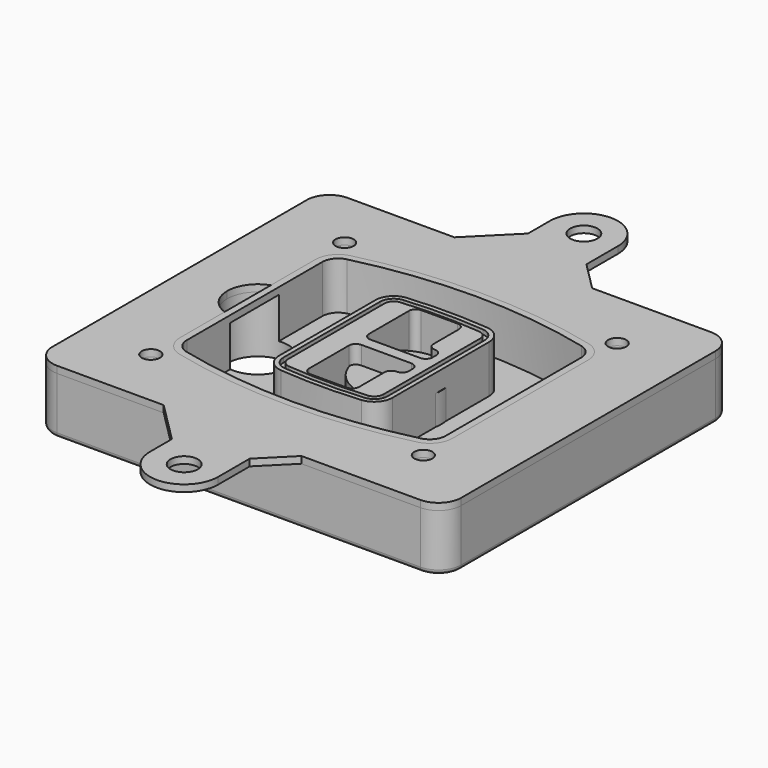
from build123d import *

# Parameters (mm, degrees)
F0_R      = 4
F1_DEPTH  = 25
F2_DEPTH  = 3
F3_DEPTH  = 18
F5_DEPTH  = 21
F6_DEPTH  = 2
F8_DEPTH  = 20
F9_DEPTH  = 16
F10_DEPTH = 25
F7_R      = 6
F7_R_2    = 4
F11_DEPTH = 6
F13_DEPTH = 9
F15_R     = 2
F16_R     = 6
F16_R_2   = 4
F17_DEPTH = 3


# Not quite as in the source:
# - a feature of the source that left no trace in its solid (it failed there, or was rolled back) is left out
# - a feature names something its author has since deleted; it is built from what else it names


with BuildPart() as f1:
    # F0 (on Top) → F1 (new body)
    with BuildSketch(Plane.XY):
        with BuildLine():
            ThreePointArc((-90, -70), (-87.0710678119, -77.0710678119), (-80, -80))
            Line((-80, -80), (80, -80))
            ThreePointArc((80, -80), (87.0710678119, -77.0710678119), (90, -70))
            Line((90, -70), (90, 70))
            ThreePointArc((90, 70), (87.0710678119, 77.0710678119), (80, 80))
            Line((80, 80), (-80, 80))
            ThreePointArc((-80, 80), (-87.0710678119, 77.0710678119), (-90, 70))
            Line((-90, 70), (-90, -70))
        make_face()
        with Locations((-60, -53.3333333333)):
            Circle(F0_R, mode=Mode.SUBTRACT)
        with Locations((60, -53.3333333333)):
            Circle(F0_R, mode=Mode.SUBTRACT)
        with Locations((-60, 53.3333333333)):
            Circle(F0_R, mode=Mode.SUBTRACT)
        with BuildLine():
            ThreePointArc((-64, 37.2990447398), (-61.0143011354, 45.9411029726), (-53.3306899286, 50.8970778549))
            ThreePointArc((-53.3306899286, 50.8970778549), (0, 57.3333333333), (53.3306899286, 50.8970778549))
            ThreePointArc((53.3306899286, 50.8970778549), (61.0143011354, 45.9411029726), (64, 37.2990447398))
            Line((64, 37.2990447398), (64, -37.2990447398))
            ThreePointArc((64, -37.2990447398), (61.0143011354, -45.9411029726), (53.3306899286, -50.8970778549))
            ThreePointArc((53.3306899286, -50.8970778549), (0, -57.3333333333), (-53.3306899286, -50.8970778549))
            ThreePointArc((-53.3306899286, -50.8970778549), (-61.0143011354, -45.9411029726), (-64, -37.2990447398))
            Line((-64, -37.2990447398), (-64, 37.2990447398))
        make_face(mode=Mode.SUBTRACT)
        with Locations((60, 53.3333333333)):
            Circle(F0_R, mode=Mode.SUBTRACT)
        with BuildLine():
            ThreePointArc((53.3306899286, 50.8970778549), (0, 57.3333333333), (-53.3306899286, 50.8970778549))
            ThreePointArc((-53.3306899286, 50.8970778549), (-61.0143011354, 45.9411029726), (-64, 37.2990447398))
            Line((-64, 37.2990447398), (-64, -37.2990447398))
            ThreePointArc((-64, -37.2990447398), (-61.0143011354, -45.9411029726), (-53.3306899286, -50.8970778549))
            ThreePointArc((-53.3306899286, -50.8970778549), (0, -57.3333333333), (53.3306899286, -50.8970778549))
            ThreePointArc((53.3306899286, -50.8970778549), (61.0143011354, -45.9411029726), (64, -37.2990447398))
            Line((64, -37.2990447398), (64, 37.2990447398))
            ThreePointArc((64, 37.2990447398), (61.0143011354, 45.9411029726), (53.3306899286, 50.8970778549))
        make_face()
        with BuildLine():
            Line((-60, -37.2990447398), (-60, 37.2990447398))
            ThreePointArc((-60, 37.2990447398), (-57.8673579538, 43.4719434775), (-52.3790642347, 47.0119255363))
            ThreePointArc((-52.3790642347, 47.0119255363), (0, 53.3333333333), (52.3790642347, 47.0119255363))
            ThreePointArc((52.3790642347, 47.0119255363), (57.8673579538, 43.4719434775), (60, 37.2990447398))
            Line((60, 37.2990447398), (60, -37.2990447398))
            ThreePointArc((60, -37.2990447398), (57.8673579538, -43.4719434775), (52.3790642347, -47.0119255363))
            ThreePointArc((52.3790642347, -47.0119255363), (0, -53.3333333333), (-52.3790642347, -47.0119255363))
            ThreePointArc((-52.3790642347, -47.0119255363), (-57.8673579538, -43.4719434775), (-60, -37.2990447398))
        make_face(mode=Mode.SUBTRACT)
        with BuildLine():
            ThreePointArc((-52.3790642347, 47.0119255363), (-57.8673579538, 43.4719434775), (-60, 37.2990447398))
            Line((-60, 37.2990447398), (-60, -37.2990447398))
            ThreePointArc((-60, -37.2990447398), (-57.8673579538, -43.4719434775), (-52.3790642347, -47.0119255363))
            ThreePointArc((-52.3790642347, -47.0119255363), (0, -53.3333333333), (52.3790642347, -47.0119255363))
            ThreePointArc((52.3790642347, -47.0119255363), (57.8673579538, -43.4719434775), (60, -37.2990447398))
            Line((60, -37.2990447398), (60, 37.2990447398))
            ThreePointArc((60, 37.2990447398), (57.8673579538, 43.4719434775), (52.3790642347, 47.0119255363))
            ThreePointArc((52.3790642347, 47.0119255363), (0, 53.3333333333), (-52.3790642347, 47.0119255363))
        make_face()
        with BuildLine():
            ThreePointArc((51.6653449643, 44.0980612973), (55.5071505677, 41.6200738562), (57, 37.2990447398))
            Line((57, 37.2990447398), (57, -37.2990447398))
            ThreePointArc((57, -37.2990447398), (55.5071505677, -41.6200738562), (51.6653449643, -44.0980612973))
            ThreePointArc((51.6653449643, -44.0980612973), (0, -50.3333333333), (-51.6653449643, -44.0980612973))
            ThreePointArc((-51.6653449643, -44.0980612973), (-55.5071505677, -41.6200738562), (-57, -37.2990447398))
            Line((-57, -37.2990447398), (-57, 37.2990447398))
            ThreePointArc((-57, 37.2990447398), (-55.5071505677, 41.6200738562), (-51.6653449643, 44.0980612973))
            ThreePointArc((-51.6653449643, 44.0980612973), (0, 50.3333333333), (51.6653449643, 44.0980612973))
        make_face(mode=Mode.SUBTRACT)
        with BuildLine():
            Line((57, -37.2990447398), (57, 37.2990447398))
            ThreePointArc((57, 37.2990447398), (55.5071505677, 41.6200738562), (51.6653449643, 44.0980612973))
            ThreePointArc((51.6653449643, 44.0980612973), (0, 50.3333333333), (-51.6653449643, 44.0980612973))
            ThreePointArc((-51.6653449643, 44.0980612973), (-55.5071505677, 41.6200738562), (-57, 37.2990447398))
            Line((-57, 37.2990447398), (-57, -37.2990447398))
            ThreePointArc((-57, -37.2990447398), (-55.5071505677, -41.6200738562), (-51.6653449643, -44.0980612973))
            ThreePointArc((-51.6653449643, -44.0980612973), (0, -50.3333333333), (51.6653449643, -44.0980612973))
            ThreePointArc((51.6653449643, -44.0980612973), (55.5071505677, -41.6200738562), (57, -37.2990447398))
        make_face()
    extrude(amount=-F1_DEPTH)

    # F0 (on Top) → F2 (join)
    with BuildSketch(Plane.XY):
        with BuildLine():
            ThreePointArc((-52.3790642347, 47.0119255363), (-57.8673579538, 43.4719434775), (-60, 37.2990447398))
            Line((-60, 37.2990447398), (-60, -37.2990447398))
            ThreePointArc((-60, -37.2990447398), (-57.8673579538, -43.4719434775), (-52.3790642347, -47.0119255363))
            ThreePointArc((-52.3790642347, -47.0119255363), (0, -53.3333333333), (52.3790642347, -47.0119255363))
            ThreePointArc((52.3790642347, -47.0119255363), (57.8673579538, -43.4719434775), (60, -37.2990447398))
            Line((60, -37.2990447398), (60, 37.2990447398))
            ThreePointArc((60, 37.2990447398), (57.8673579538, 43.4719434775), (52.3790642347, 47.0119255363))
            ThreePointArc((52.3790642347, 47.0119255363), (0, 53.3333333333), (-52.3790642347, 47.0119255363))
        make_face()
        with BuildLine():
            ThreePointArc((51.6653449643, 44.0980612973), (55.5071505677, 41.6200738562), (57, 37.2990447398))
            Line((57, 37.2990447398), (57, -37.2990447398))
            ThreePointArc((57, -37.2990447398), (55.5071505677, -41.6200738562), (51.6653449643, -44.0980612973))
            ThreePointArc((51.6653449643, -44.0980612973), (0, -50.3333333333), (-51.6653449643, -44.0980612973))
            ThreePointArc((-51.6653449643, -44.0980612973), (-55.5071505677, -41.6200738562), (-57, -37.2990447398))
            Line((-57, -37.2990447398), (-57, 37.2990447398))
            ThreePointArc((-57, 37.2990447398), (-55.5071505677, 41.6200738562), (-51.6653449643, 44.0980612973))
            ThreePointArc((-51.6653449643, 44.0980612973), (0, 50.3333333333), (51.6653449643, 44.0980612973))
        make_face(mode=Mode.SUBTRACT)
    extrude(amount=F2_DEPTH)

    # F0 (on Top) → F3 (cut)
    with BuildSketch(Plane.XY):
        with BuildLine():
            Line((57, -37.2990447398), (57, 37.2990447398))
            ThreePointArc((57, 37.2990447398), (55.5071505677, 41.6200738562), (51.6653449643, 44.0980612973))
            ThreePointArc((51.6653449643, 44.0980612973), (0, 50.3333333333), (-51.6653449643, 44.0980612973))
            ThreePointArc((-51.6653449643, 44.0980612973), (-55.5071505677, 41.6200738562), (-57, 37.2990447398))
            Line((-57, 37.2990447398), (-57, -37.2990447398))
            ThreePointArc((-57, -37.2990447398), (-55.5071505677, -41.6200738562), (-51.6653449643, -44.0980612973))
            ThreePointArc((-51.6653449643, -44.0980612973), (0, -50.3333333333), (51.6653449643, -44.0980612973))
            ThreePointArc((51.6653449643, -44.0980612973), (55.5071505677, -41.6200738562), (57, -37.2990447398))
        make_face()
    extrude(amount=-F3_DEPTH, mode=Mode.SUBTRACT)

    # F4 (on face) → F5 (join, through all)
    with BuildSketch(Plane.XY.offset(3)):
        with BuildLine():
            ThreePointArc((-25, -26.587695628), (-22.8992979869, -31.9912392117), (-17.7004291845, -34.5569740744))
            ThreePointArc((-17.7004291845, -34.5569740744), (0, -35.3333333333), (17.7004291845, -34.5569740744))
            ThreePointArc((17.7004291845, -34.5569740744), (22.8992979869, -31.9912392117), (25, -26.587695628))
            Line((25, -26.587695628), (25, 26.587695628))
            ThreePointArc((25, 26.587695628), (22.8992979869, 31.9912392117), (17.7004291845, 34.5569740744))
            ThreePointArc((17.7004291845, 34.5569740744), (0, 35.3333333333), (-17.7004291845, 34.5569740744))
            ThreePointArc((-17.7004291845, 34.5569740744), (-22.8992979869, 31.9912392117), (-25, 26.587695628))
            Line((-25, 26.587695628), (-25, -26.587695628))
        make_face()
        with BuildLine():
            ThreePointArc((17.5253218884, 32.5646544628), (21.4244734902, 30.6403533158), (23, 26.587695628))
            Line((23, 26.587695628), (23, -26.587695628))
            ThreePointArc((23, -26.587695628), (21.4244734902, -30.6403533158), (17.5253218884, -32.5646544628))
            ThreePointArc((17.5253218884, -32.5646544628), (0, -33.3333333333), (-17.5253218884, -32.5646544628))
            ThreePointArc((-17.5253218884, -32.5646544628), (-21.4244734902, -30.6403533158), (-23, -26.587695628))
            Line((-23, -26.587695628), (-23, 26.587695628))
            ThreePointArc((-23, 26.587695628), (-21.4244734902, 30.6403533158), (-17.5253218884, 32.5646544628))
            ThreePointArc((-17.5253218884, 32.5646544628), (0, 33.3333333333), (17.5253218884, 32.5646544628))
        make_face(mode=Mode.SUBTRACT)
        with BuildLine():
            Line((23, -26.587695628), (23, 26.587695628))
            ThreePointArc((23, 26.587695628), (21.4244734902, 30.6403533158), (17.5253218884, 32.5646544628))
            ThreePointArc((17.5253218884, 32.5646544628), (0, 33.3333333333), (-17.5253218884, 32.5646544628))
            ThreePointArc((-17.5253218884, 32.5646544628), (-21.4244734902, 30.6403533158), (-23, 26.587695628))
            Line((-23, 26.587695628), (-23, -26.587695628))
            ThreePointArc((-23, -26.587695628), (-21.4244734902, -30.6403533158), (-17.5253218884, -32.5646544628))
            ThreePointArc((-17.5253218884, -32.5646544628), (0, -33.3333333333), (17.5253218884, -32.5646544628))
            ThreePointArc((17.5253218884, -32.5646544628), (21.4244734902, -30.6403533158), (23, -26.587695628))
        make_face()
        with BuildLine():
            ThreePointArc((17.3502145923, 30.5723348512), (19.9496489934, 29.2894674198), (21, 26.587695628))
            Line((21, 26.587695628), (21, -26.587695628))
            ThreePointArc((21, -26.587695628), (19.9496489934, -29.2894674198), (17.3502145923, -30.5723348512))
            ThreePointArc((17.3502145923, -30.5723348512), (0, -31.3333333333), (-17.3502145923, -30.5723348512))
            ThreePointArc((-17.3502145923, -30.5723348512), (-19.9496489934, -29.2894674198), (-21, -26.587695628))
            Line((-21, -26.587695628), (-21, 26.587695628))
            ThreePointArc((-21, 26.587695628), (-19.9496489934, 29.2894674198), (-17.3502145923, 30.5723348512))
            ThreePointArc((-17.3502145923, 30.5723348512), (0, 31.3333333333), (17.3502145923, 30.5723348512))
        make_face(mode=Mode.SUBTRACT)
        with BuildLine():
            Line((21, -26.587695628), (21, 26.587695628))
            ThreePointArc((21, 26.587695628), (19.9496489934, 29.2894674198), (17.3502145923, 30.5723348512))
            ThreePointArc((17.3502145923, 30.5723348512), (0, 31.3333333333), (-17.3502145923, 30.5723348512))
            ThreePointArc((-17.3502145923, 30.5723348512), (-19.9496489934, 29.2894674198), (-21, 26.587695628))
            Line((-21, 26.587695628), (-21, -26.587695628))
            ThreePointArc((-21, -26.587695628), (-19.9496489934, -29.2894674198), (-17.3502145923, -30.5723348512))
            ThreePointArc((-17.3502145923, -30.5723348512), (0, -31.3333333333), (17.3502145923, -30.5723348512))
            ThreePointArc((17.3502145923, -30.5723348512), (19.9496489934, -29.2894674198), (21, -26.587695628))
        make_face()
        with BuildLine():
            Line((-8, -2.5), (14, -2.5))
            ThreePointArc((14, -2.5), (16.1213203436, -3.3786796564), (17, -5.5))
            Line((17, -5.5), (17, -7.5))
            ThreePointArc((17, -7.5), (16.1213203436, -9.6213203436), (14, -10.5))
            ThreePointArc((14, -10.5), (11.8786796564, -11.3786796564), (11, -13.5))
            Line((11, -13.5), (11, -27.5))
            ThreePointArc((11, -27.5), (10.1213203436, -29.6213203436), (8, -30.5))
            Line((8, -30.5), (-8, -30.5))
            ThreePointArc((-8, -30.5), (-10.1213203436, -29.6213203436), (-11, -27.5))
            Line((-11, -27.5), (-11, -5.5))
            ThreePointArc((-11, -5.5), (-10.1213203436, -3.3786796564), (-8, -2.5))
        make_face(mode=Mode.SUBTRACT)
        with BuildLine():
            ThreePointArc((-8, 2.5), (-10.1213203436, 3.3786796564), (-11, 5.5))
            Line((-11, 5.5), (-11, 27.5))
            ThreePointArc((-11, 27.5), (-10.1213203436, 29.6213203436), (-8, 30.5))
            Line((-8, 30.5), (8, 30.5))
            ThreePointArc((8, 30.5), (10.1213203436, 29.6213203436), (11, 27.5))
            Line((11, 27.5), (11, 13.5))
            ThreePointArc((11, 13.5), (11.8786796564, 11.3786796564), (14, 10.5))
            ThreePointArc((14, 10.5), (16.1213203436, 9.6213203436), (17, 7.5))
            Line((17, 7.5), (17, 5.5))
            ThreePointArc((17, 5.5), (16.1213203436, 3.3786796564), (14, 2.5))
            Line((14, 2.5), (-8, 2.5))
        make_face(mode=Mode.SUBTRACT)
    extrude(amount=-F5_DEPTH)

    # F4 (on face) → F6 (cut)
    with BuildSketch(Plane.XY.offset(3)):
        with BuildLine():
            Line((23, -26.587695628), (23, 26.587695628))
            ThreePointArc((23, 26.587695628), (21.4244734902, 30.6403533158), (17.5253218884, 32.5646544628))
            ThreePointArc((17.5253218884, 32.5646544628), (0, 33.3333333333), (-17.5253218884, 32.5646544628))
            ThreePointArc((-17.5253218884, 32.5646544628), (-21.4244734902, 30.6403533158), (-23, 26.587695628))
            Line((-23, 26.587695628), (-23, -26.587695628))
            ThreePointArc((-23, -26.587695628), (-21.4244734902, -30.6403533158), (-17.5253218884, -32.5646544628))
            ThreePointArc((-17.5253218884, -32.5646544628), (0, -33.3333333333), (17.5253218884, -32.5646544628))
            ThreePointArc((17.5253218884, -32.5646544628), (21.4244734902, -30.6403533158), (23, -26.587695628))
        make_face()
        with BuildLine():
            ThreePointArc((17.3502145923, 30.5723348512), (19.9496489934, 29.2894674198), (21, 26.587695628))
            Line((21, 26.587695628), (21, -26.587695628))
            ThreePointArc((21, -26.587695628), (19.9496489934, -29.2894674198), (17.3502145923, -30.5723348512))
            ThreePointArc((17.3502145923, -30.5723348512), (0, -31.3333333333), (-17.3502145923, -30.5723348512))
            ThreePointArc((-17.3502145923, -30.5723348512), (-19.9496489934, -29.2894674198), (-21, -26.587695628))
            Line((-21, -26.587695628), (-21, 26.587695628))
            ThreePointArc((-21, 26.587695628), (-19.9496489934, 29.2894674198), (-17.3502145923, 30.5723348512))
            ThreePointArc((-17.3502145923, 30.5723348512), (0, 31.3333333333), (17.3502145923, 30.5723348512))
        make_face(mode=Mode.SUBTRACT)
    extrude(amount=-F6_DEPTH, mode=Mode.SUBTRACT)

    # F7 (on face) → F8 (join)
    with BuildSketch(Plane(origin=(0, 0, -25), x_dir=(1, 0, 0), z_dir=(0, 0, -1))):
        with BuildLine():
            ThreePointArc((-6.71157564, 0), (6.7567035675, 13.4682792075), (20.224982775, 0))
            Line((20.224982775, 0), (25.224982775, 0))
            ThreePointArc((25.224982775, 0), (6.7567035675, 18.4682792075), (-11.71157564, 0))
            Line((-11.71157564, 0), (-6.71157564, 0))
        make_face()
        with BuildLine():
            Line((-6.71157564, 0), (20.224982775, 0))
            ThreePointArc((20.224982775, 0), (6.7567035675, 13.4682792075), (-6.71157564, 0))
        make_face()
        with BuildLine():
            ThreePointArc((-6.71157564, 0), (6.7567035675, -13.4682792075), (20.224982775, 0))
            Line((20.224982775, 0), (-6.71157564, 0))
        make_face()
        with BuildLine():
            Line((25.224982775, 0), (20.224982775, 0))
            ThreePointArc((20.224982775, 0), (6.7567035675, -13.4682792075), (-6.71157564, 0))
            Line((-6.71157564, 0), (-11.71157564, 0))
            ThreePointArc((-11.71157564, 0), (6.7567035675, -18.4682792075), (25.224982775, 0))
        make_face()
    extrude(amount=-F8_DEPTH)

    # F7 (on face) → F9 (cut)
    with BuildSketch(Plane(origin=(0, 0, -25), x_dir=(1, 0, 0), z_dir=(0, 0, -1))):
        with BuildLine():
            Line((-6.71157564, 0), (20.224982775, 0))
            ThreePointArc((20.224982775, 0), (6.7567035675, 13.4682792075), (-6.71157564, 0))
        make_face()
        with BuildLine():
            ThreePointArc((-6.71157564, 0), (6.7567035675, -13.4682792075), (20.224982775, 0))
            Line((20.224982775, 0), (-6.71157564, 0))
        make_face()
    extrude(amount=-F9_DEPTH, mode=Mode.SUBTRACT)

    # F7 (on face) → F10 (cut)
    with BuildSketch(Plane(origin=(0, 0, -25), x_dir=(1, 0, 0), z_dir=(0, 0, -1))):
        with BuildLine():
            Line((-69.0318229325, 0), (-42.0952645175, 0))
            ThreePointArc((-42.0952645175, 0), (-55.563543725, 13.4682792075), (-69.0318229325, 0))
        make_face()
        with BuildLine():
            ThreePointArc((-69.0318229325, 0), (-55.563543725, -13.4682792075), (-42.0952645175, 0))
            Line((-42.0952645175, 0), (-69.0318229325, 0))
        make_face()
    extrude(amount=-F10_DEPTH, mode=Mode.SUBTRACT)

    # F7 (on face) → F11 (cut)
    with BuildSketch(Plane(origin=(0, 0, -25), x_dir=(1, 0, 0), z_dir=(0, 0, -1))):
        with Locations((60, -53.3333333333)):
            Circle(F7_R)
        with Locations((60, -53.3333333333)):
            Circle(F7_R_2, mode=Mode.SUBTRACT)
        with Locations((-60, -53.3333333333)):
            Circle(F7_R)
        with Locations((-60, -53.3333333333)):
            Circle(F7_R_2, mode=Mode.SUBTRACT)
        with Locations((-60, 53.3333333333)):
            Circle(F7_R)
        with Locations((-60, 53.3333333333)):
            Circle(F7_R_2, mode=Mode.SUBTRACT)
        with Locations((60, 53.3333333333)):
            Circle(F7_R)
        with Locations((60, 53.3333333333)):
            Circle(F7_R_2, mode=Mode.SUBTRACT)
    extrude(amount=-F11_DEPTH, mode=Mode.SUBTRACT)

    # F12 (on face) → F13 (cut, through all)
    with BuildSketch(Plane(origin=(0, 0, -9), x_dir=(1, 0, 0), z_dir=(0, 0, -1))):
        with BuildLine():
            ThreePointArc((20.224982775, 0), (20.1663399806, 1.2554664788), (19.9909222755, 2.5))
            Line((19.9909222755, 2.5), (14, 2.5))
            ThreePointArc((14, 2.5), (16.1213203436, 3.3786796564), (17, 5.5))
            Line((17, 5.5), (17, 7.5))
            ThreePointArc((17, 7.5), (16.1213203436, 9.6213203436), (14, 10.5))
            ThreePointArc((14, 10.5), (12.1627255951, 11.1284134507), (11.0951631559, 12.750384826))
            ThreePointArc((11.0951631559, 12.750384826), (11.0476113807, 12.7664660322), (11, 12.7823698976))
            Line((11, 12.7823698976), (11, -12.7823698976))
            ThreePointArc((11, -12.7823698976), (11.0476113807, -12.7664660322), (11.0951631559, -12.750384826))
            ThreePointArc((11.0951631559, -12.750384826), (12.1627255951, -11.1284134507), (14, -10.5))
            ThreePointArc((14, -10.5), (16.1213203436, -9.6213203436), (17, -7.5))
            Line((17, -7.5), (17, -5.5))
            ThreePointArc((17, -5.5), (16.1213203436, -3.3786796564), (14, -2.5))
            Line((14, -2.5), (19.9909222755, -2.5))
            ThreePointArc((19.9909222755, -2.5), (20.1663399806, -1.2554664788), (20.224982775, 0))
        make_face()
    extrude(amount=F13_DEPTH, mode=Mode.SUBTRACT)

    # F15
    f15_edges = [f1.edges().sort_by_distance(p)[0] for p in [
        (0, -80, -25),
        (-87.071068, -77.071068, -25),
        (-90, 0, -25),
        (-87.071068, 77.071068, -25),
        (87.071068, -77.071068, -25),
        (0, 80, -25),
        (90, 0, -25),
        (87.071068, 77.071068, -25),
    ]]
    fillet(f15_edges, radius=F15_R)


with BuildPart() as f17:
    # F16 (on face) → F17 (new body, through all)
    with BuildSketch(Plane.XY):
        with BuildLine():
            Line((27.6571478513, -80), (-33, -80))
            Line((-33, -80), (-15, -98))
            Line((-15, -98), (-15, -110))
            ThreePointArc((-15, -110), (0, -125), (15, -110))
            Line((15, -110), (15, -92.6571478513))
            Line((15, -92.6571478513), (27.6571478513, -80))
        make_face()
        with Locations((0, -110)):
            Circle(F16_R, mode=Mode.SUBTRACT)
        with BuildLine():
            ThreePointArc((15, 110), (0, 125), (-15, 110))
            Line((-15, 110), (-15, 98))
            Line((-15, 98), (-33, 80))
            Line((-33, 80), (27.6571478513, 80))
            Line((27.6571478513, 80), (15, 92.6571478513))
            Line((15, 92.6571478513), (15, 110))
        make_face()
        with Locations((0, 110)):
            Circle(F16_R, mode=Mode.SUBTRACT)
        with BuildLine():
            Line((27.6571478513, 80), (-33, 80))
            Line((-33, 80), (-80, 80))
            ThreePointArc((-80, 80), (-87.0710678119, 77.0710678119), (-90, 70))
            Line((-90, 70), (-90, -70))
            ThreePointArc((-90, -70), (-87.0710678119, -77.0710678119), (-80, -80))
            Line((-80, -80), (-33, -80))
            Line((-33, -80), (27.6571478513, -80))
            Line((27.6571478513, -80), (80, -80))
            ThreePointArc((80, -80), (87.0710678119, -77.0710678119), (90, -70))
            Line((90, -70), (90, 70))
            ThreePointArc((90, 70), (87.0710678119, 77.0710678119), (80, 80))
            Line((80, 80), (27.6571478513, 80))
        make_face()
        with Locations((-60, -53.3333333333)):
            Circle(F16_R_2, mode=Mode.SUBTRACT)
        with Locations((60, -53.3333333333)):
            Circle(F16_R_2, mode=Mode.SUBTRACT)
        with Locations((-60, 53.3333333333)):
            Circle(F16_R_2, mode=Mode.SUBTRACT)
        with BuildLine():
            ThreePointArc((-60, 37.2990447398), (-57.8673579538, 43.4719434775), (-52.3790642347, 47.0119255363))
            ThreePointArc((-52.3790642347, 47.0119255363), (0, 53.3333333333), (52.3790642347, 47.0119255363))
            ThreePointArc((52.3790642347, 47.0119255363), (57.8673579538, 43.4719434775), (60, 37.2990447398))
            Line((60, 37.2990447398), (60, -37.2990447398))
            ThreePointArc((60, -37.2990447398), (57.8673579538, -43.4719434775), (52.3790642347, -47.0119255363))
            ThreePointArc((52.3790642347, -47.0119255363), (0, -53.3333333333), (-52.3790642347, -47.0119255363))
            ThreePointArc((-52.3790642347, -47.0119255363), (-57.8673579538, -43.4719434775), (-60, -37.2990447398))
            Line((-60, -37.2990447398), (-60, -12.7166190685))
            ThreePointArc((-60, -12.7166190685), (-66.5441169481, -7.798817635), (-69.0318229325, 0))
            ThreePointArc((-69.0318229325, 0), (-66.5441169481, 7.798817635), (-60, 12.7166190685))
            Line((-60, 12.7166190685), (-60, 37.2990447398))
        make_face(mode=Mode.SUBTRACT)
        with Locations((60, 53.3333333333)):
            Circle(F16_R_2, mode=Mode.SUBTRACT)
    extrude(amount=F17_DEPTH)


solid = Compound([f1.part, f17.part])
